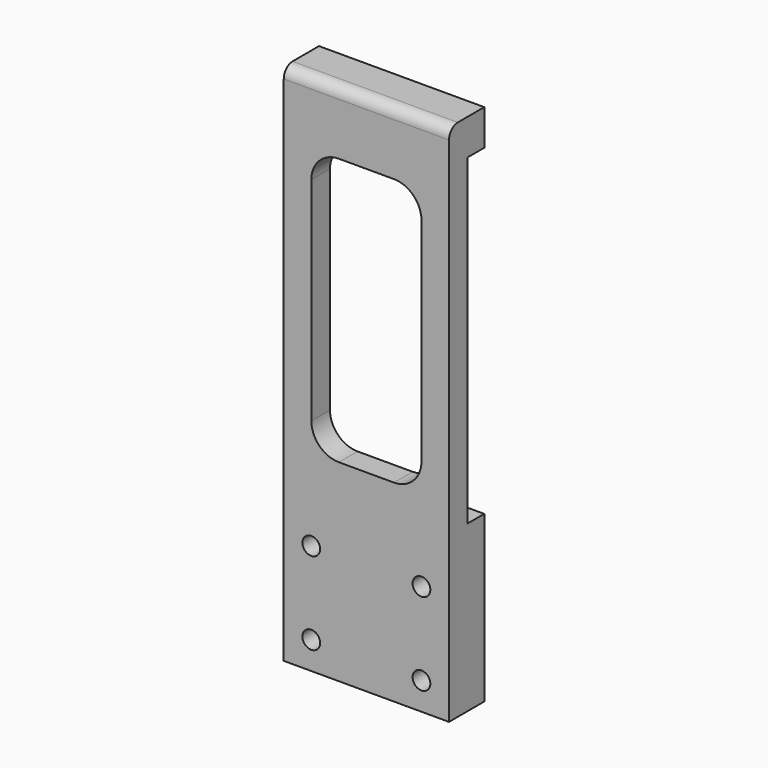
from build123d import *

# Parameters (mm, degrees)
F1_DEPTH = 25
F2_R     = 1.6101418037
F3_DEPTH = 25
F5_DEPTH = 70
F6_W     = 3.75
F6_H     = 58.5
F7_DEPTH = 30.001
F8_W     = 20
F8_H     = 48.5
F9_DEPTH = 25
F10_R    = 5
F11_R    = 2


with BuildPart() as f1:
    # F0 (on Top) → F1 (new body)
    with BuildSketch(Plane.XY):
        with BuildLine():
            Line((15, 4), (3.9, 4))
            ThreePointArc((3.9, 4), (0, 0.1), (-3.9, 4))
            Line((-3.9, 4), (-15, 4))
            Line((-15, 4), (-15, -4))
            Line((-15, -4), (15, -4))
            Line((15, -4), (15, 4))
        make_face()
    extrude(amount=F1_DEPTH)

    # F2 (on face) → F3 (cut)
    with BuildSketch(Plane.XZ.offset(4)):
        with Locations((-10, 20)):
            Circle(F2_R)
        with Locations((-10, 5)):
            Circle(F2_R)
        with Locations((10, 20)):
            Circle(F2_R)
        with Locations((10, 5)):
            Circle(F2_R)
    extrude(amount=-F3_DEPTH, mode=Mode.SUBTRACT)

    # F4 (on face) → F5 (join)
    with BuildSketch(Plane.XY.offset(25)):
        with BuildLine():
            Line((-15, 4), (-15, -4))
            Line((-15, -4), (15, -4))
            Line((15, -4), (15, 4))
            Line((15, 4), (3.9, 4))
            ThreePointArc((3.9, 4), (0, 0.1), (-3.9, 4))
            Line((-3.9, 4), (-15, 4))
        make_face()
        with BuildLine():
            Line((3.9, 4), (-3.9, 4))
            ThreePointArc((-3.9, 4), (0, 0.1), (3.9, 4))
        make_face()
    extrude(amount=F5_DEPTH)

    # F6 (on face) → F7 (cut, through all)
    with BuildSketch(Plane(origin=(-15, 0, 0), x_dir=(0, -1, 0), z_dir=(-1, 0, 0))):
        with Locations((-2.125, 59.25)):
            Rectangle(F6_W, F6_H)
    extrude(amount=-F7_DEPTH, mode=Mode.SUBTRACT)

    # F8 (on face) → F9 (cut)
    with BuildSketch(Plane(origin=(0, 0.25, 0), x_dir=(-1, 0, 0), z_dir=(0, 1, 0))):
        with Locations((0, 59.25)):
            Rectangle(F8_W, F8_H)
    extrude(amount=-F9_DEPTH, mode=Mode.SUBTRACT)

    # F10
    f10_edges = [f1.edges().sort_by_distance(p)[0] for p in [
        (10, -1.875, 35),
        (-10, -1.875, 83.5),
        (-10, -1.875, 35),
        (10, -1.875, 83.5),
    ]]
    fillet(f10_edges, radius=F10_R)

    # F11
    f11_edges = [f1.edges().sort_by_distance(p)[0] for p in [
        (0, -4, 95),
    ]]
    fillet(f11_edges, radius=F11_R)


solid = f1.part
